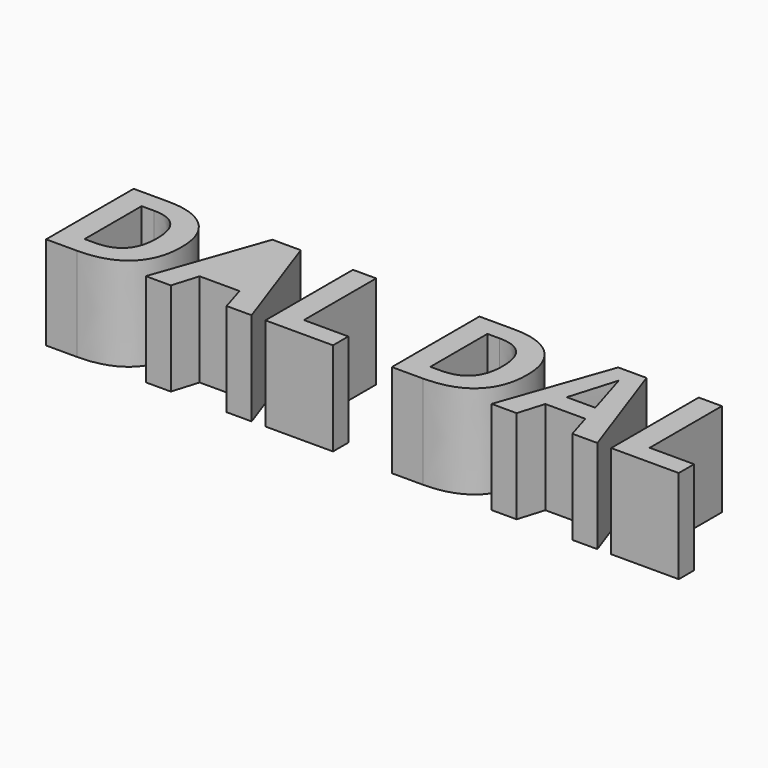
from build123d import *

# Parameters (mm, degrees)
F0_TEXT_SIZE = 41.6562607926
F1_DEPTH     = 25.4


# Not quite as in the source:
# - Text() gives the source's letters only with a copy of the font that has no kerning and outlines rounded to 1/6400 em; it was checked with that copy


with BuildPart() as f1:
    # F0 (on Top) → F1 (new body)
    with BuildSketch(Plane.XY):
        with Locations((-66.2929991546, -29.9925077707)):
            Text('DAL DAL', F0_TEXT_SIZE, font='Open Sans', font_style=FontStyle.BOLD, text_align=(TextAlign.LEFT, TextAlign.BOTTOM))
        with BuildLine():
            Line((-24.9166163643, -17.6258053479), (-17.1711553731, -17.6258053479))
            add(Edge.make_bspline(
                [(-17.1711553731, -17.6258053479), (-20.1586903269, -8.0058126211), (-20.5362001903, -6.7431072158)],
                knots=[0, 0, 0, 1, 1, 1], degree=2))
            add(Edge.make_bspline(
                [(-20.5362001903, -6.7431072158), (-20.9137100537, -5.4804018105), (-21.0764298224, -4.7514172467)],
                knots=[0, 0, 0, 1, 1, 1], degree=2))
            add(Edge.make_bspline(
                [(-21.0764298224, -4.7514172467), (-21.7468352696, -7.3549335462), (-24.9166163643, -17.6258053479)],
                knots=[0, 0, 0, 1, 1, 1], degree=2))
        make_face()
    extrude(amount=F1_DEPTH)


solid = f1.part
